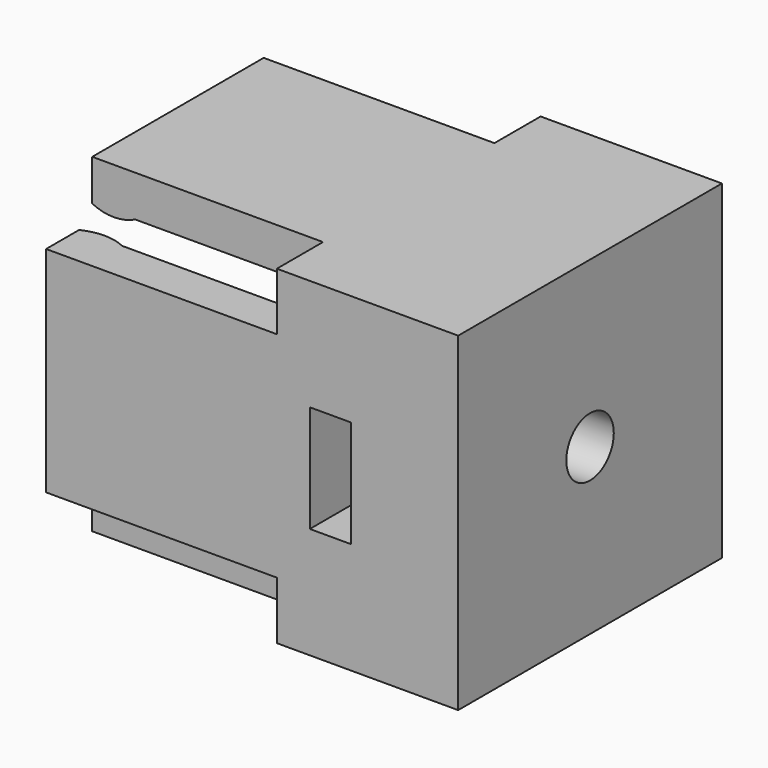
from build123d import *

# Parameters (mm, degrees)
F0_W            = 20
F0_H            = 20
F0_R            = 1.8
F1_DEPTH        = 11
F2_W            = 13
F2_H            = 2.5
F2_W_2          = 2.5
F2_H_2          = 13
F3_DEPTH        = 14
F2_R            = 2.5
F2_R_2          = 1.8
F4_DEPTH        = 1
F5_W            = 2.5
F5_H            = 6.5
F6_DEPTH        = 25
F8_DEPTH        = 13
F8_COPIES_COUNT = 4


# Not quite as in the source:
# - a pattern or mirror of a feature is missing from the dataset's text; its kind, count and spacing are read off the source's solid


with BuildPart() as f1:
    # F0 (on Right) → F1 (new body)
    with BuildSketch(Plane.YZ):
        Rectangle(F0_W, F0_H)
        Circle(F0_R, mode=Mode.SUBTRACT)
    extrude(amount=-F1_DEPTH)

    # F2 (on face) → F3 (join)
    with BuildSketch(Plane(origin=(-11, 0, 0), x_dir=(0, -1, 0), z_dir=(-1, 0, 0))):
        with Locations((0, -8.75)):
            Rectangle(F2_W, F2_H)
        with Locations((8.75, 0)):
            Rectangle(F2_W_2, F2_H_2)
        with Locations((-8.75, 0)):
            Rectangle(F2_W_2, F2_H_2)
        with Locations((0, 8.75)):
            Rectangle(F2_W, F2_H)
    extrude(amount=F3_DEPTH)

    # F2 (on face) → F4 (cut)
    with BuildSketch(Plane(origin=(-11, 0, 0), x_dir=(0, -1, 0), z_dir=(-1, 0, 0))):
        Circle(F2_R)
        Circle(F2_R_2, mode=Mode.SUBTRACT)
    extrude(amount=-F4_DEPTH, mode=Mode.SUBTRACT)

    # F5 (on face) → F6 (cut)
    with BuildSketch(Plane.XZ.offset(10)):
        with Locations((-7.75, 0)):
            Rectangle(F5_W, F5_H)
    extrude(amount=-F6_DEPTH, mode=Mode.SUBTRACT)

    # F7 (on face) → F8 (join, through all)
    with BuildSketch(Plane.XZ.offset(6.5)):
        with BuildLine():
            Line((-25, -7.5), (-22.3846606339, -7.5))
            ThreePointArc((-22.3846606339, -7.5), (-23.6923303169, -7.2), (-25, -7.5))
        make_face()
    f8 = extrude(amount=-F8_DEPTH)

    # F8_copies: F8 ×4 about axis
    f8_copies_axis = Axis((0, 0, 0), (1, 0, 0))
    for i in range(1, F8_COPIES_COUNT):
        add(f8.rotate(f8_copies_axis, i * 360 / F8_COPIES_COUNT))


solid = f1.part
